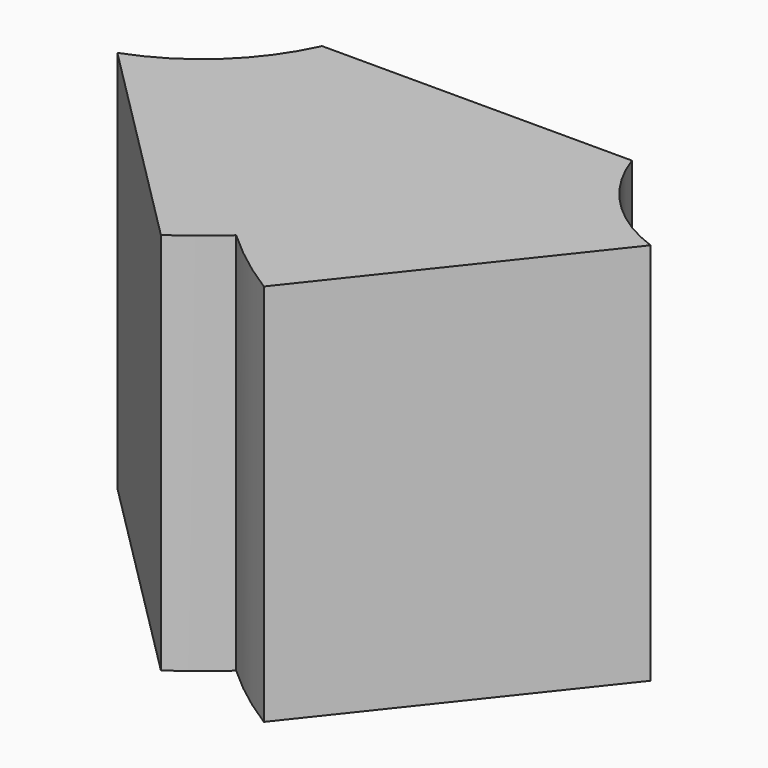
from build123d import *

# Parameters (mm, degrees)
F0_W = 76.971642673
F0_H = 95.2017754316


# Not quite as in the source:
# - a feature names something its author has since deleted; it is built from what else it names
# - the program builds the solid bodies; features that only make, move or delete a surface that nothing else refers to are left out


with BuildPart() as f2:
    # F2: sweep along a path in F1
    with BuildLine(Plane.XY) as f2_path:
        ThreePointArc((0, 0), (13.4369935077, -32.3954640503), (39.643291384, -55.703163147))
    # F0 (on Front) → F2 (sweep)
    with BuildSketch(Plane.XZ):
        Rectangle(F0_W, F0_H)
    sweep(path=f2_path.line)

    # F3: sweep along a path in F1
    with BuildLine(Plane.XY) as f3_path:
        ThreePointArc((-40.5113920569, -54.2563311756), (-14.8539477386, -31.1614707896), (0, 0))
    # F0 (on Front) → F3 (sweep)
    with BuildSketch(Plane.XZ):
        Rectangle(F0_W, F0_H)
    sweep(path=f3_path.line)


solid = f2.part
